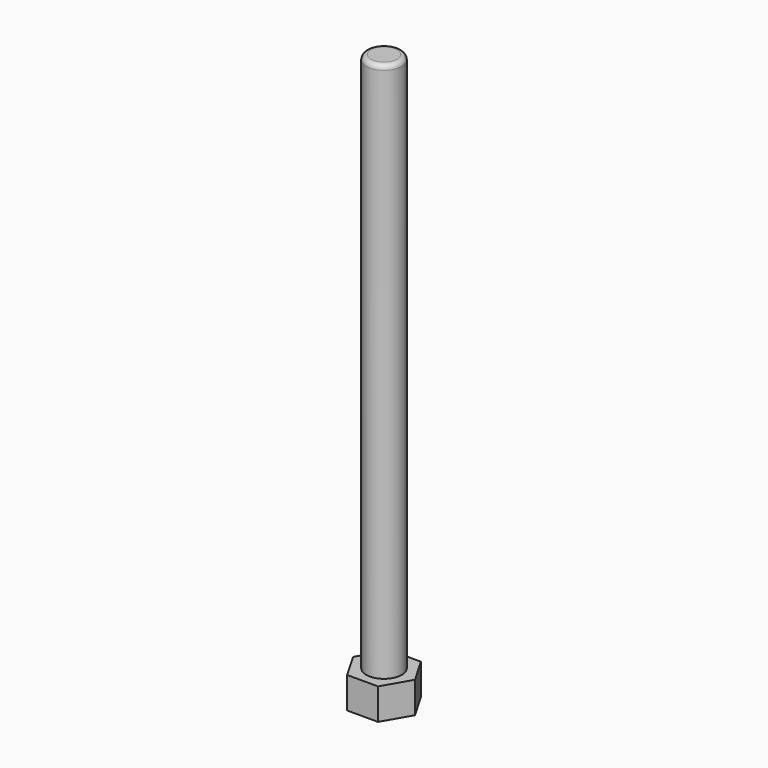
from build123d import *

# Parameters (mm, degrees)
F0_R     = 4.74599
F1_DEPTH = 152.4
F3_DEPTH = 8.334375
F4_R     = 1.27


# Not quite as in the source:
# - a length typed as a fraction of an inch, garbled in the dataset ("3 / 203.2 mm" for 3/8 in), is restored


with BuildPart() as f1:
    # F0 (on Top) → F1 (new body)
    with BuildSketch(Plane.XY):
        Circle(F0_R)
    extrude(amount=F1_DEPTH)

    # F2 (on Top) → F3 (join)
    with BuildSketch(Plane.XY):
        Polygon((-4.1244459855, -7.14375), (4.1244459855, -7.14375), (8.248891971, 0), (4.1244459855, 7.14375), (-4.1244459855, 7.14375), (-8.248891971, 0), align=None)
    extrude(amount=F3_DEPTH)

    # F4
    f4_edges = [f1.edges().sort_by_distance(p)[0] for p in [
        (-4.74599, 0, 152.4),
    ]]
    fillet(f4_edges, radius=F4_R)


solid = f1.part
